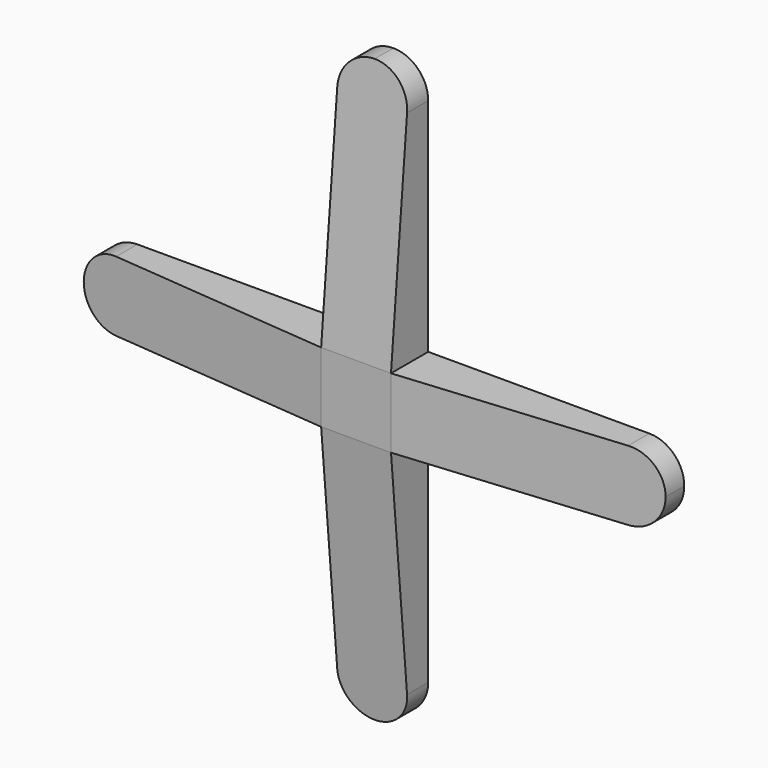
from build123d import *

# Parameters (mm, degrees)
F0_W      = 30
F0_H      = 30
F1_DEPTH  = 20
F5_W      = 20
F5_H      = 30
F6_DEPTH  = 110
F4_W      = 30
F4_H      = 20
F7_DEPTH  = 110
F3_W      = 20
F3_H      = 30
F8_DEPTH  = 110
F2_W      = 30
F2_H      = 20
F9_DEPTH  = 110
F10_SIZE2 = 10
F10_SIZE  = 110
F11_R     = 14.99999


# Not quite as in the source:
# - a fillet or chamfer is up to 0.001 mm smaller than in the source, because OpenCascade refuses the exact size


with BuildPart() as f1:
    # F0 (on Front) → F1 (new body)
    with BuildSketch(Plane.XZ):
        Rectangle(F0_W, F0_H)
    extrude(amount=F1_DEPTH)

    # F5 (on face) → F6 (join)
    with BuildSketch(Plane.YZ.offset(15)):
        with Locations((-10, 0)):
            Rectangle(F5_W, F5_H)
    extrude(amount=F6_DEPTH)

    # F4 (on face) → F7 (join)
    with BuildSketch(Plane.XY.offset(15)):
        with Locations((0, -10)):
            Rectangle(F4_W, F4_H)
    extrude(amount=F7_DEPTH)

    # F3 (on face) → F8 (join)
    with BuildSketch(Plane(origin=(-15, 0, 0), x_dir=(0, -1, 0), z_dir=(-1, 0, 0))):
        with Locations((10, 0)):
            Rectangle(F3_W, F3_H)
    extrude(amount=F8_DEPTH)

    # F2 (on face) → F9 (join)
    with BuildSketch(Plane(origin=(0, 0, -15), x_dir=(1, 0, 0), z_dir=(0, 0, -1))):
        with Locations((0, 10)):
            Rectangle(F2_W, F2_H)
    extrude(amount=F9_DEPTH)

    # F10
    f10_edges = [f1.edges().sort_by_distance(p)[0] for p in [
        (-125, -20, 0),
        (0, -20, -125),
        (125, -20, 0),
        (0, -20, 125),
    ]]
    f10_side = f1.faces().sort_by_distance((0, -20, 0))[0]
    chamfer(f10_edges, length=F10_SIZE, length2=F10_SIZE2, reference=f10_side)

    # F11 (radius 15 in the source; OpenCascade refuses exactly that, so slightly less here)
    f11_edges = [f1.edges().sort_by_distance(p)[0] for p in [
        (15, -5, 125),
        (-15, -5, 125),
        (-125, -5, 15),
        (-125, -5, -15),
        (-15, -5, -125),
        (15, -5, -125),
        (125, -5, -15),
        (125, -5, 15),
    ]]
    fillet(f11_edges, radius=F11_R)


solid = f1.part
